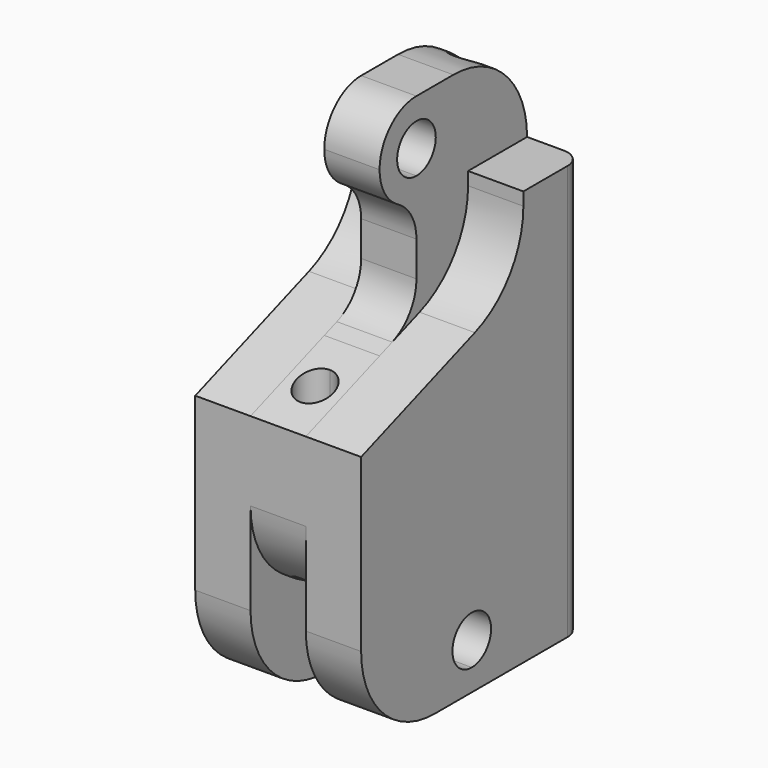
from build123d import *

# Parameters (mm, degrees)
F1_DEPTH     = 15
F3_DEPTH     = 6
F5_DEPTH     = 18
F6_R         = 10
F9_DEPTH     = 6
F10_DEPTH    = 6
F11_R        = 2
F13_DEPTH    = 6
F15_R        = 10
F18_DEPTH    = 40
F20_DEPTH    = 45
F22_DEPTH    = 6
F23_T1_DEPTH = 6


# Not quite as in the source:
# - a fillet or chamfer that OpenCascade refuses, or shapes differently, is made with other operations: its cross-section is extruded or revolved along the edge and cut away or added


with BuildPart() as f1:
    # F0 (on Front) → F1 (new body, symmetric)
    with BuildSketch(Plane.XZ):
        Polygon((9, -17.5), (9, 17.5), (3, 17.5), (3, 27.5), (-3, 27.5), (-3, 17.5), (-9, 17.5), (-9, -17.5), (-9, -27.5), (-3, -27.5), (-3, -17.5), (3, -17.5), (3, -27.5), (9, -27.5), align=None)
    extrude(amount=F1_DEPTH, both=True)

    # F2 (on face) → F3 (cut)
    with BuildSketch(Plane(origin=(-3, 0, 0), x_dir=(0, -1, 0), z_dir=(-1, 0, 0))):
        with BuildLine():
            ThreePointArc((0, 25.12), (-2.62, 22.5), (0, 19.88))
            Line((0, 19.88), (0, 25.12))
        make_face()
        with BuildLine():
            Line((0, 25.12), (0, 19.88))
            ThreePointArc((0, 19.88), (1.8526197667, 20.6473802333), (2.62, 22.5))
            ThreePointArc((2.62, 22.5), (1.8526197667, 24.3526197667), (0, 25.12))
        make_face()
    extrude(amount=-F3_DEPTH, mode=Mode.SUBTRACT)

    # F4 (on face) → F5 (cut)
    with BuildSketch(Plane(origin=(-9, 0, 0), x_dir=(0, -1, 0), z_dir=(-1, 0, 0))):
        with BuildLine():
            ThreePointArc((0, -25.12), (1.8526197667, -24.3526197667), (2.62, -22.5))
            ThreePointArc((2.62, -22.5), (-1.8526197667, -20.6473802333), (0, -25.12))
        make_face()
    extrude(amount=-F5_DEPTH, mode=Mode.SUBTRACT)

    # F6
    f6_edges = [f1.edges().sort_by_distance(p)[0] for p in [
        (0, 15, 27.5),
        (0, -15, 27.5),
        (6, -15, -27.5),
        (-6, -15, -27.5),
    ]]
    fillet(f6_edges, radius=F6_R)

    # F8 (on face) → F9 (cut)
    with BuildSketch(Plane(origin=(-9, 0, 0), x_dir=(0, -1, 0), z_dir=(-1, 0, 0))):
        with BuildLine():
            ThreePointArc((-7, 16.0872004348), (-5.1915204429, 10.3514360713), (-0.4202014333, 6.690274227))
            Line((-0.4202014333, 6.690274227), (15, 1.0777798989))
            Line((15, 1.0777798989), (15, 17.5))
            Line((15, 17.5), (-7, 17.5))
            Line((-7, 17.5), (-7, 16.0872004348))
        make_face()
    extrude(amount=-F9_DEPTH, mode=Mode.SUBTRACT)

    # F7 (on face) → F10 (cut)
    with BuildSketch(Plane.YZ.offset(9)):
        with BuildLine():
            Line((7, 17.5), (-15, 17.5))
            Line((-15, 17.5), (-15, 1.07778))
            Line((-15, 1.07778), (0.4202014333, 6.6902743281))
            ThreePointArc((0.4202014333, 6.6902743281), (5.1915204429, 10.3514361724), (7, 16.087200536))
            Line((7, 16.087200536), (7, 17.5))
        make_face()
    extrude(amount=-F10_DEPTH, mode=Mode.SUBTRACT)

    # F11
    f11_edges = [f1.edges().sort_by_distance(p)[0] for p in [
        (9, 15, -5),
        (-9, 15, -5),
    ]]
    fillet(f11_edges, radius=F11_R)

    # F12 (on face) → F13 (cut)
    with BuildSketch(Plane(origin=(-3, 0, 0), x_dir=(0, -1, 0), z_dir=(-1, 0, 0))):
        with BuildLine():
            Line((5, 27.5), (0, 27.5))
            ThreePointArc((0, 27.5), (3.5355339059, 26.0355339059), (5, 22.5))
            Line((5, 22.5), (5, 4.7174822415))
            Line((5, 4.7174822415), (15, 1.0777798989))
            Line((15, 1.0777798989), (15, 17.5))
            ThreePointArc((15, 17.5), (12.0710678119, 24.5710678119), (5, 27.5))
        make_face()
    extrude(amount=-F13_DEPTH, mode=Mode.SUBTRACT)

    # F15
    f15_edges = [f1.edges().sort_by_distance(p)[0] for p in [
        (0, -15, -17.5),
    ]]
    fillet(f15_edges, radius=F15_R)

    # F17 (on face) → F18 (cut)
    with BuildSketch(Plane.XY.offset(22.5)):
        with BuildLine():
            ThreePointArc((2, -10), (1.4142135624, -8.5857864376), (0, -8))
            Line((0, -8), (0, -12))
            ThreePointArc((0, -12), (1.4142135624, -11.4142135624), (2, -10))
        make_face()
        with BuildLine():
            Line((0, -12), (0, -8))
            ThreePointArc((0, -8), (-2, -10), (0, -12))
        make_face()
    extrude(amount=-F18_DEPTH, mode=Mode.SUBTRACT)

    # F19 (on face) → F20 (cut)
    with BuildSketch(Plane(origin=(0, 0, -17.5), x_dir=(1, 0, 0), z_dir=(0, 0, -1))):
        with BuildLine():
            ThreePointArc((0, -9), (-2, -11), (0, -13))
            Line((0, -13), (0, -11))
            Line((0, -11), (0, -9))
        make_face()
        with BuildLine():
            Line((0, -11), (0, -13))
            ThreePointArc((0, -13), (1.4142135624, -12.4142135624), (2, -11))
            ThreePointArc((2, -11), (1.4142135624, -9.5857864376), (0, -9))
            Line((0, -9), (0, -11))
        make_face()
    extrude(amount=-F20_DEPTH, mode=Mode.SUBTRACT)

    # F21 (on face) → F22 (cut)
    with BuildSketch(Plane(origin=(-3, 0, 0), x_dir=(0, -1, 0), z_dir=(-1, 0, 0))):
        with BuildLine():
            ThreePointArc((5, 22.5), (3.5355339059, 18.9644660941), (0, 17.5))
            Line((0, 17.5), (0, 6.5373334129))
            Line((0, 6.5373334129), (5, 4.7174822415))
            Line((5, 4.7174822415), (5, 22.5))
        make_face()
    extrude(amount=-F22_DEPTH, mode=Mode.SUBTRACT)

    # F23: fillet of radius 5 on 2 edges, made by hand

    # F23_s2 → F23_t1 (join)
    with BuildSketch(Plane.YZ.offset(-3)):
        with BuildLine():
            ThreePointArc((-2.5, 18.1698729811), (-0.6698729811, 16.3397459622), (0, 13.8397459622))
            Line((0, 13.8397459622), (0, 17.5))
            ThreePointArc((0, 17.5), (-1.2940952255, 17.6703708686), (-2.5, 18.1698729811))
        make_face()
        with BuildLine():
            ThreePointArc((-3.2898992834, 5.3399081011), (-0.9042397786, 7.1704890233), (0, 10.038371205))
            Line((0, 10.038371205), (0, 6.5373334129))
            Line((0, 6.5373334129), (-3.2898992834, 5.3399081011))
        make_face()
    extrude(amount=F23_T1_DEPTH)


solid = f1.part
